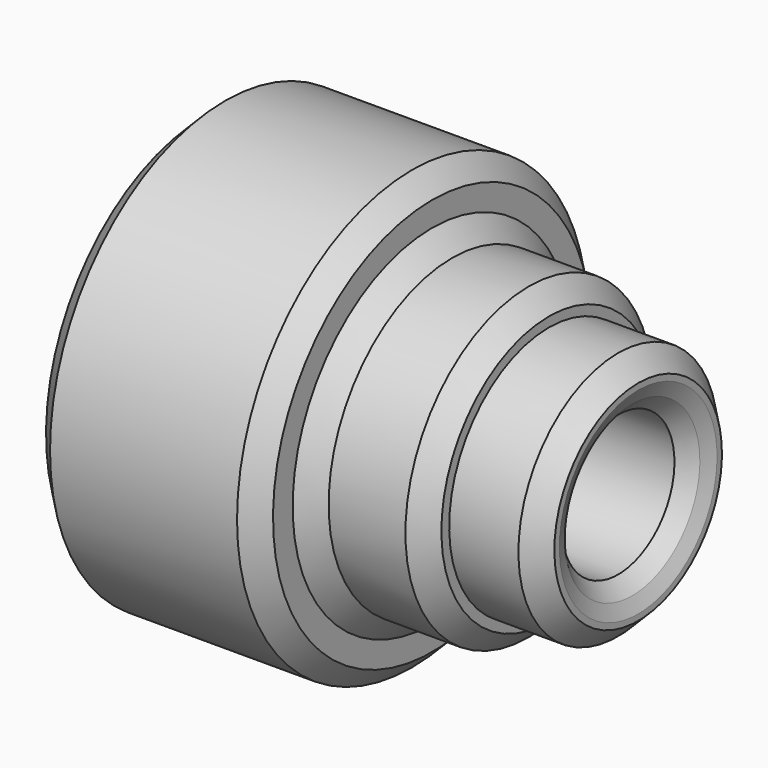
from build123d import *

# Parameters (mm, degrees)
F1_W    = 23.5887104645
F1_H    = 20.866939798
F1_W_2  = 22.3185494542
F1_H_2  = 13.6088710278
F1_W_3  = 19.2338721827
F3_SIZE = 5


# Not quite as in the source:
# - a fillet or chamfer that OpenCascade refuses, or shapes differently, is made with other operations: its cross-section is extruded or revolved along the edge and cut away or added


with BuildPart() as f2:
    # F1 (on Front) → F2 (revolve)
    with BuildSketch(Plane.XZ):
        Polygon((-13.9717748389, 54.798386991), (-70.7661360502, 54.798386991), (-70.7661360502, 17.7822578698), (-37.5604853034, 17.7822578698), (-37.5604853034, 38.6491976678), (-13.9717748389, 38.6491976678), align=None)
        Polygon((15.2419358492, 38.6491976678), (-13.9717748389, 38.6491976678), (-13.9717748389, 17.7822578698), (-37.5604853034, 17.7822578698), (-37.5604853034, 17.6008082926), (-3.9919363335, 17.6008082926), (-3.9919363335, 31.2096793205), (15.2419358492, 31.2096793205), align=None)
        with Locations((-25.7661300711, 28.2157277688)):
            Rectangle(F1_W, F1_H)
        with Locations((26.4012105763, 24.4052438065)):
            Rectangle(F1_W_2, F1_H_2)
        with Locations((5.6249997579, 24.4052438065)):
            Rectangle(F1_W_3, F1_H_2)
    revolve(axis=Axis((0.2721734345, 0, 0), (1, 0, 0)))

    # F3
    f3_edges = [f2.edges().sort_by_distance(p)[0] for p in [
        (-13.971775, 0, -54.798387),
        (-70.766136, 0, -54.798387),
        (-42.368955, 0, 54.798387),
        (37.560485, 0, -17.600808),
    ]]
    chamfer(f3_edges, length=F3_SIZE)

    # F4: chamfer of 5 on 5 edges, made by hand

    # F4_s1 → F4_t2 (revolve)
    with BuildSketch(Plane.XZ):
        Polygon((-13.9717748389, 43.6491976678), (-8.9717748389, 38.6491976678), (-13.9717748389, 38.6491976678), align=None)
    revolve(axis=Axis((-13.9717748389, 0, 0), (1, 0, 0)))

    # F4_s3 → F4_t4 (revolve, cut)
    with BuildSketch(Plane.XZ):
        Polygon((32.5604853034, 31.2096793205), (37.5604853034, 26.2096793205), (37.5604853034, 31.2096793205), align=None)
    revolve(axis=Axis((37.5604853034, 0, 0), (1, 0, 0)), mode=Mode.SUBTRACT)

    # F4_s5 → F4_t6 (revolve, cut)
    with BuildSketch(Plane.XZ):
        Polygon((36.0960192093, 21.1363421986), (37.5604853034, 24.6718761045), (37.5604853034, 22.6008082926), align=None)
    revolve(axis=Axis((37.5604853034, 0, 0), (1, 0, 0)), mode=Mode.SUBTRACT)

    # F4_s7 → F4_t8 (revolve, cut)
    with BuildSketch(Plane.XZ):
        Polygon((10.2419358492, 38.6491976678), (15.2419358492, 33.6491976678), (15.2419358492, 38.6491976678), align=None)
    revolve(axis=Axis((15.2419358492, 0, 0), (1, 0, 0)), mode=Mode.SUBTRACT)


solid = f2.part
